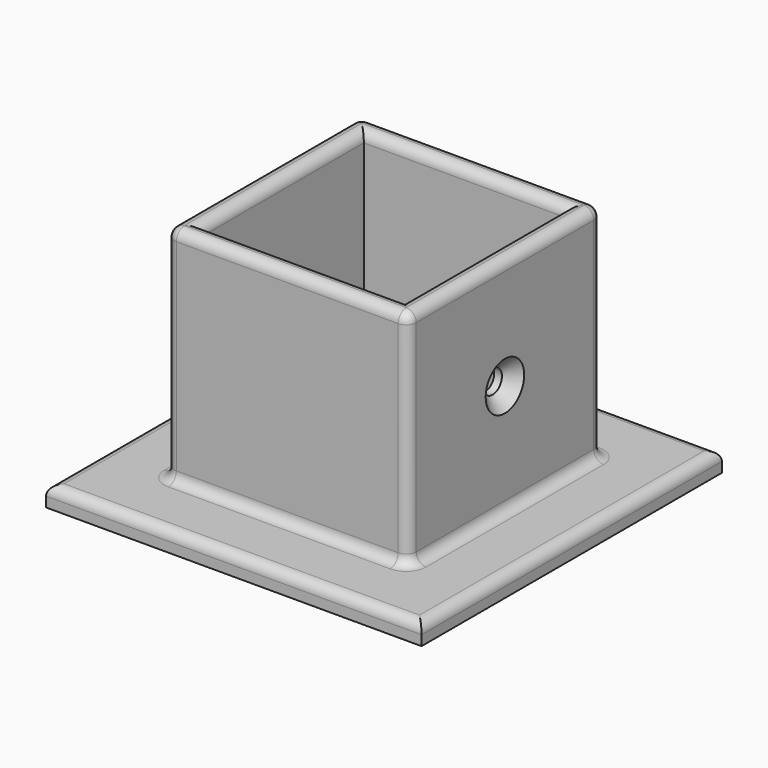
from build123d import *

# Parameters (mm, degrees)
F0_W           = 56.2
F0_H           = 56.2
F1_DEPTH       = 3
F2_W           = 36.2
F2_H           = 36.2
F2_W_2         = 30.2
F2_H_2         = 30.2
F3_DEPTH       = 33.2
F4_D           = 3.5
F4_DEPTH       = 13.5
F4_CSINK_D     = 7.2
F4_CSINK_ANGLE = 90
F4_TIP         = 1.0515060833
F5_R           = 1.49999
F7_D           = 3.5
F7_DEPTH       = 13.5
F7_CSINK_D     = 7.2
F7_CSINK_ANGLE = 90
F7_TIP         = 1.0515060833


# Not quite as in the source:
# - a fillet or chamfer is up to 0.001 mm smaller than in the source, because OpenCascade refuses the exact size
# - a feature names something its author has since deleted; it is built from what else it names


with BuildPart() as f1:
    # F0 (on Top) → F1 (new body)
    with BuildSketch(Plane.XY):
        with Locations((18.1, 18.1)):
            Rectangle(F0_W, F0_H)
    extrude(amount=F1_DEPTH)

    # F2 (on face) → F3 (join)
    with BuildSketch(Plane.XY.offset(3)):
        with Locations((18.1, 18.1)):
            Rectangle(F2_W, F2_H)
        with Locations((18.1, 18.1)):
            Rectangle(F2_W_2, F2_H_2, mode=Mode.SUBTRACT)
    extrude(amount=F3_DEPTH)

    # F4
    with Locations(Plane.XY.offset(3)):
        with Locations((18.1, 18.1)):
            CounterSinkHole(F4_D / 2, F4_CSINK_D / 2, depth=F4_DEPTH, counter_sink_angle=F4_CSINK_ANGLE)
            with Locations((0, 0, -(F4_DEPTH + F4_TIP / 2))):  # 118° drill point
                Cone(0, F4_D / 2, F4_TIP, mode=Mode.SUBTRACT)

    # F5 (radius 1.5 in the source; OpenCascade refuses exactly that, so slightly less here)
    f5_edges = [f1.edges().sort_by_distance(p)[0] for p in [
        (33.2, 18.1, 36.2),
        (18.1, 3, 36.2),
        (18.1, 0, 3),
        (18.1, 33.2, 36.2),
        (3, 18.1, 36.2),
        (0, 18.1, 36.2),
        (18.1, 36.2, 36.2),
        (36.2, 18.1, 36.2),
        (18.1, 0, 36.2),
        (36.2, 0, 19.6),
        (0, 0, 19.6),
        (0, 18.1, 3),
        (18.1, 36.2, 3),
        (36.2, 36.2, 19.6),
        (0, 36.2, 19.6),
        (18.1, 46.2, 3),
        (-10, 18.1, 3),
        (18.1, -10, 3),
        (46.2, 18.1, 3),
        (36.2, 18.1, 3),
    ]]
    fillet(f5_edges, radius=F5_R)

    # F7
    with Locations(Plane.YZ.offset(36.2)):
        with Locations((18.1, 19.6)):
            CounterSinkHole(F7_D / 2, F7_CSINK_D / 2, depth=F7_DEPTH, counter_sink_angle=F7_CSINK_ANGLE)
            with Locations((0, 0, -(F7_DEPTH + F7_TIP / 2))):  # 118° drill point
                Cone(0, F7_D / 2, F7_TIP, mode=Mode.SUBTRACT)


solid = f1.part
